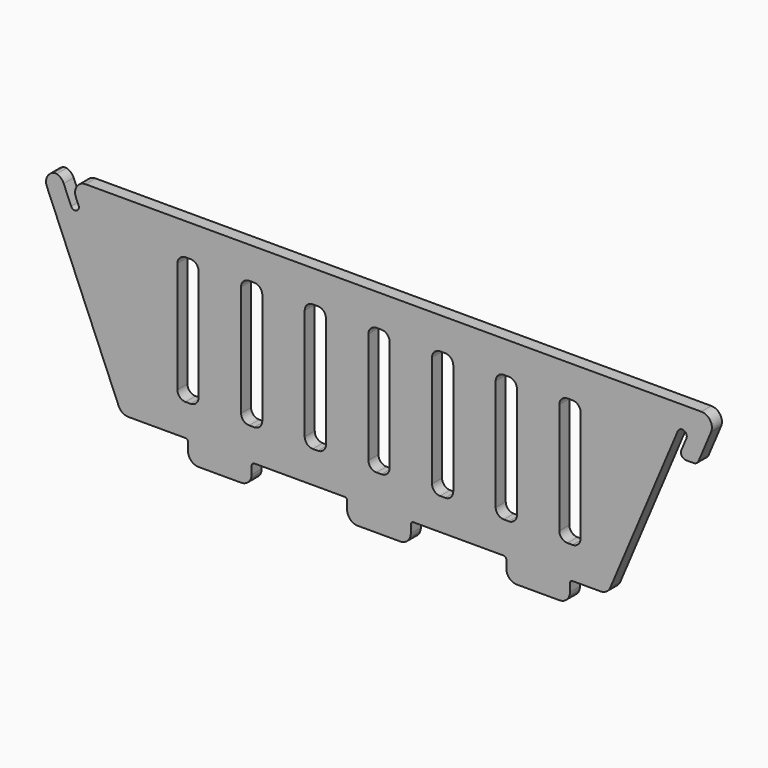
from build123d import *

# Parameters (mm, degrees)
F1_DEPTH = 15


# Not quite as in the source:
# - ends of sketch curves that miss each other by under 0.0002 mm in the source are joined


with BuildPart() as f1:
    # F0 (on Front) → F1 (new body)
    with BuildSketch(Plane.XZ):
        with BuildLine():
            Line((152.4, -104.775), (152.4, -114.3))
            ThreePointArc((152.4, -114.3), (156.1197438789, -123.2802561211), (165.1, -127))
            Line((165.1, -127), (215.9, -127))
            ThreePointArc((215.9, -127), (224.8802561211, -123.2802561211), (228.6, -114.3))
            Line((228.6, -114.3), (228.6, -104.775))
            ThreePointArc((228.6, -104.775), (229.5299359697, -102.5299359697), (231.775, -101.6))
            Line((231.775, -101.6), (265.179556, -101.6))
            ThreePointArc((265.179556, -101.6), (272.1974896575, -99.4848291048), (276.8777652022, -93.8438751462))
            Line((276.8777652022, -93.8438751462), (357.711629, 97.4253068))
            ThreePointArc((357.711629, 97.4253068), (365.0341452454, 100.3972108736), (368.0060482736, 93.0746921546))
            Line((368.0060482736, 93.0746921546), (361.9191644, 78.6719534))
            ThreePointArc((361.9191644, 78.6719534), (362.4758586154, 72.6910380462), (367.7682764, 69.85))
            Line((367.7682764, 69.85), (376.592338, 69.85))
            ThreePointArc((376.592338, 69.85), (380.1013055832, 70.9075859478), (382.4414433059, 73.7280640946))
            Line((382.4414433059, 73.7280640946), (397.4984938, 109.3561186))
            ThreePointArc((397.4984938, 109.3561186), (396.3851270368, 121.3179295371), (385.8002952, 127))
            Line((385.8002952, 127), (-351.0556098, 127))
            ThreePointArc((-351.0556098, 127), (-361.6404416368, 121.3179295371), (-362.7538151531, 109.356115746))
            Line((-362.7538151531, 109.356115746), (-359.6258238, 101.9546856))
            ThreePointArc((-359.6258238, 101.9546856), (-362.1924804362, 95.6306809293), (-368.5164757001, 98.1973326577))
            Line((-368.5164757001, 98.1973326577), (-377.411107, 119.2438814))
            ThreePointArc((-377.411107, 119.2438814), (-380.76124871, 123.8707639235), (-385.8003211895, 126.5613398156))
            ThreePointArc((-385.8003211895, 126.5613398156), (-387.4548258, 126.780671), (-389.1093307052, 126.5613409078))
            ThreePointArc((-389.1093307052, 126.5613409078), (-397.2156200075, 119.8660524106), (-397.4985259531, 109.356115746))
            Line((-397.4985259531, 109.356115746), (-311.6224908, -93.8438814))
            ThreePointArc((-311.6224908, -93.8438814), (-306.9422004575, -99.4848291048), (-299.9242668, -101.6))
            Line((-299.9242668, -101.6), (-231.775, -101.6))
            ThreePointArc((-231.775, -101.6), (-229.5299359697, -102.5299359697), (-228.6, -104.775))
            Line((-228.6, -104.775), (-228.6, -114.3))
            ThreePointArc((-228.6, -114.3), (-224.8802561211, -123.2802561211), (-215.9, -127))
            Line((-215.9, -127), (-165.1, -127))
            ThreePointArc((-165.1, -127), (-156.1197438789, -123.2802561211), (-152.4, -114.3))
            Line((-152.4, -114.3), (-152.4, -104.775))
            ThreePointArc((-152.4, -104.775), (-151.4700640303, -102.5299359697), (-149.225, -101.6))
            Line((-149.225, -101.6), (-41.275, -101.6))
            ThreePointArc((-41.275, -101.6), (-39.0299359697, -102.5299359697), (-38.1, -104.775))
            Line((-38.1, -104.775), (-38.1, -114.3))
            ThreePointArc((-38.1, -114.3), (-34.3802561211, -123.2802561211), (-25.4, -127))
            Line((-25.4, -127), (25.4, -127))
            ThreePointArc((25.4, -127), (34.3802561211, -123.2802561211), (38.1, -114.3))
            Line((38.1, -114.3), (38.1, -104.775))
            ThreePointArc((38.1, -104.775), (39.0299359697, -102.5299359697), (41.275, -101.6))
            Line((41.275, -101.6), (149.225, -101.6))
            ThreePointArc((149.225, -101.6), (151.4700640303, -102.5299359697), (152.4, -104.775))
        make_face()
        with BuildLine():
            ThreePointArc((-215.9, -53.848), (-218.727005348, -60.672994652), (-225.552, -63.5))
            Line((-225.552, -63.5), (-231.648, -63.5))
            ThreePointArc((-231.648, -63.5), (-238.472994652, -60.672994652), (-241.3, -53.848))
            Line((-241.3, -53.848), (-241.3, 79.248))
            ThreePointArc((-241.3, 79.248), (-238.472994652, 86.072994652), (-231.648, 88.9))
            Line((-231.648, 88.9), (-225.552, 88.9))
            ThreePointArc((-225.552, 88.9), (-218.727005348, 86.072994652), (-215.9, 79.248))
            Line((-215.9, 79.248), (-215.9, -53.848))
        make_face(mode=Mode.SUBTRACT)
        with BuildLine():
            ThreePointArc((-139.7, -53.848), (-142.527005348, -60.672994652), (-149.352, -63.5))
            Line((-149.352, -63.5), (-155.448, -63.5))
            ThreePointArc((-155.448, -63.5), (-162.272994652, -60.672994652), (-165.1, -53.848))
            Line((-165.1, -53.848), (-165.1, 79.248))
            ThreePointArc((-165.1, 79.248), (-162.272994652, 86.072994652), (-155.448, 88.9))
            Line((-155.448, 88.9), (-149.352, 88.9))
            ThreePointArc((-149.352, 88.9), (-142.527005348, 86.072994652), (-139.7, 79.248))
            Line((-139.7, 79.248), (-139.7, -53.848))
        make_face(mode=Mode.SUBTRACT)
        with BuildLine():
            ThreePointArc((-63.5, -53.848), (-66.327005348, -60.672994652), (-73.152, -63.5))
            Line((-73.152, -63.5), (-79.248, -63.5))
            ThreePointArc((-79.248, -63.5), (-86.072994652, -60.672994652), (-88.9, -53.848))
            Line((-88.9, -53.848), (-88.9, 79.248))
            ThreePointArc((-88.9, 79.248), (-86.072994652, 86.072994652), (-79.248, 88.9))
            Line((-79.248, 88.9), (-73.152, 88.9))
            ThreePointArc((-73.152, 88.9), (-66.327005348, 86.072994652), (-63.5, 79.248))
            Line((-63.5, 79.248), (-63.5, -53.848))
        make_face(mode=Mode.SUBTRACT)
        with BuildLine():
            ThreePointArc((12.7, -53.848), (9.872994652, -60.672994652), (3.048, -63.5))
            Line((3.048, -63.5), (-3.048, -63.5))
            ThreePointArc((-3.048, -63.5), (-9.872994652, -60.672994652), (-12.7, -53.848))
            Line((-12.7, -53.848), (-12.7, 79.248))
            ThreePointArc((-12.7, 79.248), (-9.872994652, 86.072994652), (-3.048, 88.9))
            Line((-3.048, 88.9), (3.048, 88.9))
            ThreePointArc((3.048, 88.9), (9.872994652, 86.072994652), (12.7, 79.248))
            Line((12.7, 79.248), (12.7, -53.848))
        make_face(mode=Mode.SUBTRACT)
        with BuildLine():
            ThreePointArc((88.9, -53.848), (86.072994652, -60.672994652), (79.248, -63.5))
            Line((79.248, -63.5), (73.152, -63.5))
            ThreePointArc((73.152, -63.5), (66.327005348, -60.672994652), (63.5, -53.848))
            Line((63.5, -53.848), (63.5, 79.248))
            ThreePointArc((63.5, 79.248), (66.327005348, 86.072994652), (73.152, 88.9))
            Line((73.152, 88.9), (79.248, 88.9))
            ThreePointArc((79.248, 88.9), (86.072994652, 86.072994652), (88.9, 79.248))
            Line((88.9, 79.248), (88.9, -53.848))
        make_face(mode=Mode.SUBTRACT)
        with BuildLine():
            ThreePointArc((165.1, -53.848), (162.272994652, -60.672994652), (155.448, -63.5))
            Line((155.448, -63.5), (149.352, -63.5))
            ThreePointArc((149.352, -63.5), (142.527005348, -60.672994652), (139.7, -53.848))
            Line((139.7, -53.848), (139.7, 79.248))
            ThreePointArc((139.7, 79.248), (142.527005348, 86.072994652), (149.352, 88.9))
            Line((149.352, 88.9), (155.448, 88.9))
            ThreePointArc((155.448, 88.9), (162.272994652, 86.072994652), (165.1, 79.248))
            Line((165.1, 79.248), (165.1, -53.848))
        make_face(mode=Mode.SUBTRACT)
        with BuildLine():
            ThreePointArc((241.3, -53.848), (238.472994652, -60.672994652), (231.648, -63.5))
            Line((231.648, -63.5), (225.552, -63.5))
            ThreePointArc((225.552, -63.5), (218.727005348, -60.672994652), (215.9, -53.848))
            Line((215.9, -53.848), (215.9, 79.248))
            ThreePointArc((215.9, 79.248), (218.727005348, 86.072994652), (225.552, 88.9))
            Line((225.552, 88.9), (231.648, 88.9))
            ThreePointArc((231.648, 88.9), (238.472994652, 86.072994652), (241.3, 79.248))
            Line((241.3, 79.248), (241.3, -53.848))
        make_face(mode=Mode.SUBTRACT)
    extrude(amount=F1_DEPTH)


solid = f1.part
